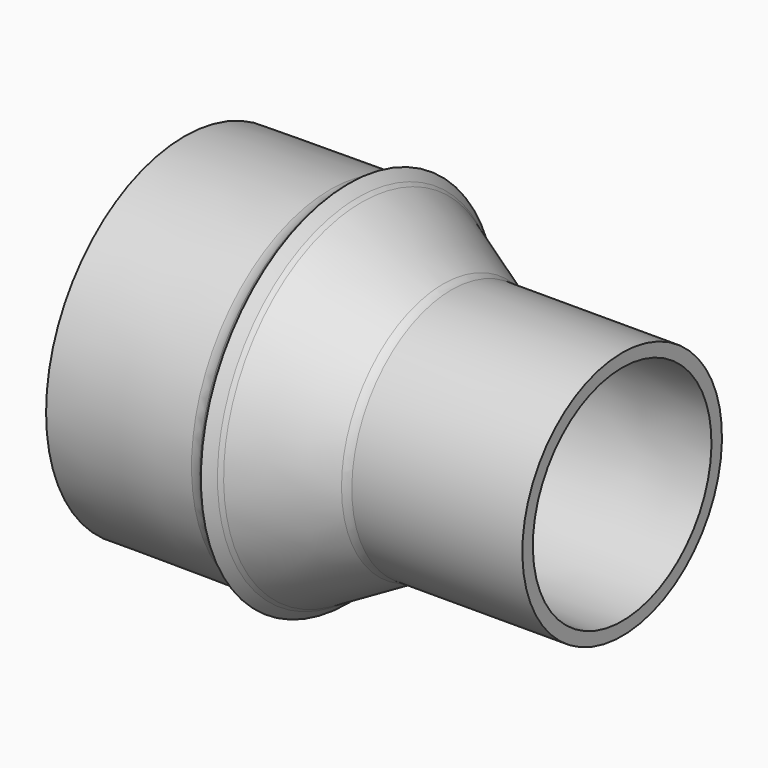
from build123d import *

# Parameters (mm, degrees)
F3_R = 5.08


# Not quite as in the source:
# - a variable given as a bare number and used for a length is read in inches; the dataset says mm whatever the document's units were


with BuildPart() as f2:
    # F1 (on Front) → F2 (revolve)
    with BuildSketch(Plane.XZ):
        Polygon((-25.4, 46.355), (0, 31.75), (50.8, 32.385), (50.8, 36.195), (0, 36.195), (-25.4, 50.38725), (-28.575, 53.56225), (-31.75, 50.38725), (-76.2, 50.165), (-76.2, 46.355), align=None)
    revolve(axis=Axis((-24.3991323134, 0, 0), (-1, 0, 0)))

    # F3
    f3_edges = [f2.edges().sort_by_distance(p)[0] for p in [
        (-25.4, 0, -46.355),
        (0, 0, -31.75),
        (0, 0, -36.195),
        (-31.75, 0, -50.38725),
        (-25.4, 0, -50.38725),
    ]]
    fillet(f3_edges, radius=F3_R)


solid = f2.part
